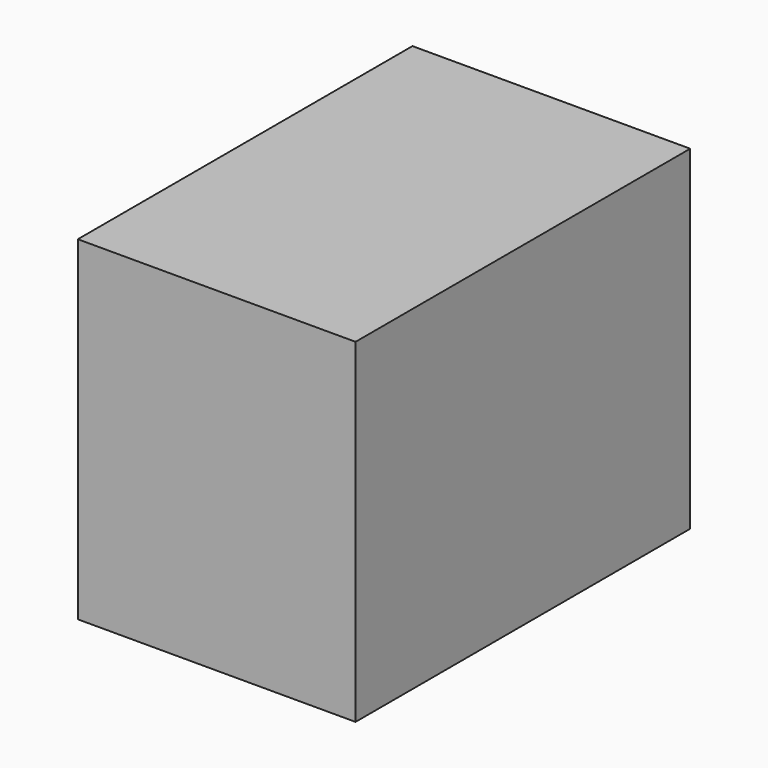
from build123d import *

# Parameters (mm, degrees)
F0_W     = 16.6
F0_H     = 20
F2_DEPTH = 25


# Not quite as in the source:
# - a feature of the source that left no trace in its solid (it failed there, or was rolled back) is left out


with BuildPart() as f2:
    # F0 (on Front) → F2 (new body)
    with BuildSketch(Plane.XZ):
        with Locations((-26.5731932595, 28.1553536495)):
            Rectangle(F0_W, F0_H)
    extrude(amount=F2_DEPTH)


solid = f2.part
